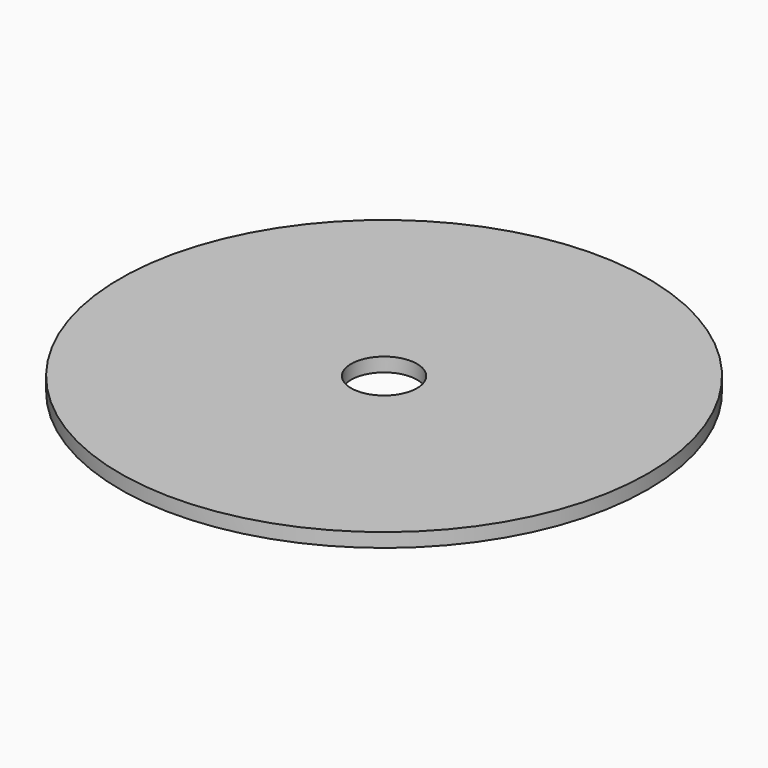
from build123d import *

# Parameters (mm, degrees)
F0_R     = 60.000134
F0_R_2   = 7.493
F1_DEPTH = 3.175


# Not quite as in the source:
# - a length typed as a fraction of an inch, garbled in the dataset ("3 / 203.2 mm" for 3/8 in), is restored


with BuildPart() as f1:
    # F0 (on Top) → F1 (new body)
    with BuildSketch(Plane.XY):
        Circle(F0_R)
        Circle(F0_R_2, mode=Mode.SUBTRACT)
    extrude(amount=F1_DEPTH)


solid = f1.part
